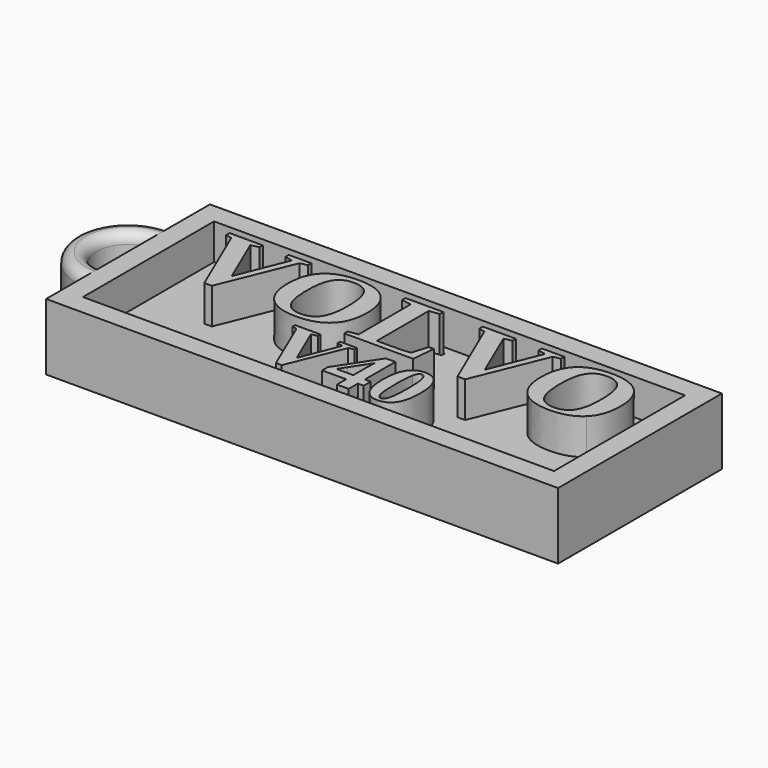
from build123d import *

# Parameters (mm, degrees)
F1_DEPTH = 3
F2_DEPTH = 3.5
F3_R     = 0.99999


# Not quite as in the source:
# - a fillet or chamfer is up to 0.001 mm smaller than in the source, because OpenCascade refuses the exact size


with BuildPart() as f1:
    # F0 (on Top) → F1 (new body)
    with BuildSketch(Plane.XY):
        Polygon((25, -10), (25, 10), (0, 10), (0, 8), (23, 8), (23, -8), (0, -8), (0, -10), align=None)
        Polygon((0, 8), (0, 10), (-25, 10), (-25, 5.1), (-25, 3.1), (-25, -3.1), (-25, -5.1), (-25, -10), (0, -10), (0, -8), (-23, -8), (-23, 8), align=None)
        with BuildLine():
            Line((23, 8), (0, 8))
            Line((0, 8), (0, 7.2330922616))
            Line((0, 7.2330922616), (0.1773994991, 7.2330922616))
            Line((0.1773994991, 7.2330922616), (0.1773994991, 6.8265888868))
            Line((0.1773994991, 6.8265888868), (0, 6.8041054881))
            Line((0, 6.8041054881), (0, 0.3510614427))
            Line((0, 0.3510614427), (0.544678864, 0.3510614427))
            add(Edge.make_bspline(
                [(0.544678864, 0.3510614427), (1.7320966167, 0.3510614427), (2.2901473023, 0.4633847436)],
                knots=[0, 0, 0, 1, 1, 1], degree=2))
            Line((2.2901473023, 0.4633847436), (2.7465721442, 2.0180818613))
            Line((2.7465721442, 2.0180818613), (3.2475697245, 2.0180818613))
            Line((3.2475697245, 2.0180818613), (3.0354034894, -0.2390816146))
            Line((3.0354034894, -0.2390816146), (0, -0.2390816146))
            Line((0, -0.2390816146), (0, -3.5619589872))
            Line((0, -3.5619589872), (1.3642210542, -1.4834557912))
            Line((1.3642210542, -1.4834557912), (2.2953560595, -1.4834557912))
            Line((2.2953560595, -1.4834557912), (2.2953560595, -5.197168661))
            Line((2.2953560595, -5.197168661), (2.861074711, -5.197168661))
            Line((2.861074711, -5.197168661), (2.861074711, -6.0646941529))
            Line((2.861074711, -6.0646941529), (2.2953560595, -6.0646941529))
            Line((2.2953560595, -6.0646941529), (2.2953560595, -7.1853043046))
            Line((2.2953560595, -7.1853043046), (1.1571517871, -7.1853043046))
            Line((1.1571517871, -7.1853043046), (1.1571517871, -6.0646941529))
            Line((1.1571517871, -6.0646941529), (0, -6.0646941529))
            Line((0, -6.0646941529), (0, -8))
            Line((0, -8), (23, -8))
            Line((23, -8), (23, 8))
        make_face()
        with BuildLine():
            add(Edge.make_bspline(
                [(6.5578701571, -2.1628595305), (7.0227609628, -2.9004592076), (7.0227609628, -4.3255829875)],
                knots=[0, 0, 0, 1, 1, 1], degree=2))
            add(Edge.make_bspline(
                [(7.0227609628, -4.3255829875), (7.0227609628, -7.2705681205), (5.1618443461, -7.2705681205)],
                knots=[0, 0, 0, 1, 1, 1], degree=2))
            add(Edge.make_bspline(
                [(5.1618443461, -7.2705681205), (4.2658975823, -7.2705681205), (3.8091271401, -6.5174044134)],
                knots=[0, 0, 0, 1, 1, 1], degree=2))
            add(Edge.make_bspline(
                [(3.8091271401, -6.5174044134), (3.3523566978, -5.7642407064), (3.3523566978, -4.3255829875)],
                knots=[0, 0, 0, 1, 1, 1], degree=2))
            add(Edge.make_bspline(
                [(3.3523566978, -4.3255829875), (3.3523566978, -2.9180533284), (3.8091271401, -2.1716565908)],
                knots=[0, 0, 0, 1, 1, 1], degree=2))
            add(Edge.make_bspline(
                [(3.8091271401, -2.1716565908), (4.2658975823, -1.4252598533), (5.1956791937, -1.4252598533)],
                knots=[0, 0, 0, 1, 1, 1], degree=2))
            add(Edge.make_bspline(
                [(5.1956791937, -1.4252598533), (6.0929793514, -1.4252598533), (6.5578701571, -2.1628595305)],
                knots=[0, 0, 0, 1, 1, 1], degree=2))
        make_face(mode=Mode.SUBTRACT)
        Polygon((9.6393004203, 7.2330922616), (11.8394107908, 7.2330922616), (11.8394107908, 6.8265888868), (11.131595704, 6.675041576), (8.2450651611, -0.4120238398), (7.5051577026, -0.4120238398), (4.4688627584, 6.675041576), (3.8555418771, 6.8265888868), (3.8555418771, 7.2330922616), (7.1040030564, 7.2330922616), (7.1040030564, 6.8265888868), (6.3284374071, 6.675041576), (8.4304877531, 1.7773890735), (10.3916882455, 6.675041576), (9.6393004203, 6.8265888868), align=None, mode=Mode.SUBTRACT)
        with BuildLine():
            add(Edge.make_bspline(
                [(13.5224773953, 0.6238466021), (12.5258309632, 1.5990981197), (12.5258309632, 3.5050284164)],
                knots=[0, 0, 0, 1, 1, 1], degree=2))
            add(Edge.make_bspline(
                [(12.5258309632, 3.5050284164), (12.5258309632, 7.3168890099), (16.4090079382, 7.3168890099)],
                knots=[0, 0, 0, 1, 1, 1], degree=2))
            add(Edge.make_bspline(
                [(16.4090079382, 7.3168890099), (18.3256356922, 7.3168890099), (19.3062359384, 6.3496605852)],
                knots=[0, 0, 0, 1, 1, 1], degree=2))
            add(Edge.make_bspline(
                [(19.3062359384, 6.3496605852), (20.2868361846, 5.3824321605), (20.2868361846, 3.5050284164)],
                knots=[0, 0, 0, 1, 1, 1], degree=2))
            add(Edge.make_bspline(
                [(20.2868361846, 3.5050284164), (20.2868361846, 1.6044468483), (19.2946470264, 0.6265209664)],
                knots=[0, 0, 0, 1, 1, 1], degree=2))
            add(Edge.make_bspline(
                [(19.2946470264, 0.6265209664), (18.3024578681, -0.3514049155), (16.4090079382, -0.3514049155)],
                knots=[0, 0, 0, 1, 1, 1], degree=2))
            add(Edge.make_bspline(
                [(16.4090079382, -0.3514049155), (14.5191238273, -0.3514049155), (13.5224773953, 0.6238466021)],
                knots=[0, 0, 0, 1, 1, 1], degree=2))
        make_face(mode=Mode.SUBTRACT)
        Polygon((0, 7.2330922616), (0, 8), (-23, 8), (-23, -8), (0, -8), (0, -6.0646941529), (-1.1896332408, -6.0646941529), (-1.1896332408, -5.3744632623), (0, -3.5619589872), (0, -0.2390816146), (-3.6897312901, -0.2390816146), (-3.6897312901, 0.1674217602), (-2.7305259583, 0.318969071), (-2.7305259583, 6.6803903046), (-3.6825996519, 6.8265888868), (-3.6825996519, 7.2330922616), align=None)
        Polygon((-3.0762643416, -1.513230457), (-1.4061762652, -1.513230457), (-1.4061762652, -1.8218042669), (-1.9434736447, -1.9368427487), (-4.1346183737, -7.3165835132), (-4.6962768435, -7.3165835132), (-7.0011066603, -1.9368427487), (-7.466674163, -1.8218042669), (-7.466674163, -1.513230457), (-5.0007904717, -1.513230457), (-5.0007904717, -1.8218042669), (-5.5895168195, -1.9368427487), (-3.9938654078, -5.6546158003), (-2.5051321145, -1.9368427487), (-3.0762643416, -1.8218042669), align=None, mode=Mode.SUBTRACT)
        Polygon((-15.0878719701, 7.2330922616), (-12.8877615995, 7.2330922616), (-12.8877615995, 6.8265888868), (-13.5955766863, 6.675041576), (-16.4821072293, -0.4120238398), (-17.2220146878, -0.4120238398), (-20.258309632, 6.675041576), (-20.8716305132, 6.8265888868), (-20.8716305132, 7.2330922616), (-17.623169334, 7.2330922616), (-17.623169334, 6.8265888868), (-18.3987349832, 6.675041576), (-16.2966846373, 1.7773890735), (-14.3354841448, 6.675041576), (-15.0878719701, 6.8265888868), align=None, mode=Mode.SUBTRACT)
        with BuildLine():
            add(Edge.make_bspline(
                [(-11.2046949951, 0.6238466021), (-12.2013414272, 1.5990981197), (-12.2013414272, 3.5050284164)],
                knots=[0, 0, 0, 1, 1, 1], degree=2))
            add(Edge.make_bspline(
                [(-12.2013414272, 3.5050284164), (-12.2013414272, 7.3168890099), (-8.3181644522, 7.3168890099)],
                knots=[0, 0, 0, 1, 1, 1], degree=2))
            add(Edge.make_bspline(
                [(-8.3181644522, 7.3168890099), (-6.4015366982, 7.3168890099), (-5.420936452, 6.3496605852)],
                knots=[0, 0, 0, 1, 1, 1], degree=2))
            add(Edge.make_bspline(
                [(-5.420936452, 6.3496605852), (-4.4403362058, 5.3824321605), (-4.4403362058, 3.5050284164)],
                knots=[0, 0, 0, 1, 1, 1], degree=2))
            add(Edge.make_bspline(
                [(-4.4403362058, 3.5050284164), (-4.4403362058, 1.6044468483), (-5.432525364, 0.6265209664)],
                knots=[0, 0, 0, 1, 1, 1], degree=2))
            add(Edge.make_bspline(
                [(-5.432525364, 0.6265209664), (-6.4247145222, -0.3514049155), (-8.3181644522, -0.3514049155)],
                knots=[0, 0, 0, 1, 1, 1], degree=2))
            add(Edge.make_bspline(
                [(-8.3181644522, -0.3514049155), (-10.2080485631, -0.3514049155), (-11.2046949951, 0.6238466021)],
                knots=[0, 0, 0, 1, 1, 1], degree=2))
        make_face(mode=Mode.SUBTRACT)
        with BuildLine():
            Line((-25, 3.1), (-25, 5.1))
            ThreePointArc((-25, 5.1), (-30.1, 0), (-25, -5.1))
            Line((-25, -5.1), (-25, -3.1))
            ThreePointArc((-25, -3.1), (-28.1, 0), (-25, 3.1))
        make_face()
        Polygon((0, 6.8041054881), (0, 7.2330922616), (-3.6825996519, 7.2330922616), (-3.6825996519, 6.8265888868), (-2.7305259583, 6.6803903046), (-2.7305259583, 0.318969071), (-3.6897312901, 0.1674217602), (-3.6897312901, -0.2390816146), (0, -0.2390816146), (0, 0.3510614427), (-0.9761429724, 0.3510614427), (-0.9761429724, 6.6803903046), align=None)
        Polygon((0, 0.3510614427), (0, 6.8041054881), (-0.9761429724, 6.6803903046), (-0.9761429724, 0.3510614427), align=None)
        Polygon((-1.1896332408, -6.0646941529), (0, -6.0646941529), (0, -5.197168661), (-0.488575199, -5.197168661), (0, -4.4515723469), (0, -3.5619589872), (-1.1896332408, -5.3744632623), align=None)
        with BuildLine():
            Line((0, -5.197168661), (0, -6.0646941529))
            Line((0, -6.0646941529), (1.1571517871, -6.0646941529))
            Line((1.1571517871, -6.0646941529), (1.1571517871, -7.1853043046))
            Line((1.1571517871, -7.1853043046), (2.2953560595, -7.1853043046))
            Line((2.2953560595, -7.1853043046), (2.2953560595, -6.0646941529))
            Line((2.2953560595, -6.0646941529), (2.861074711, -6.0646941529))
            Line((2.861074711, -6.0646941529), (2.861074711, -5.197168661))
            Line((2.861074711, -5.197168661), (2.2953560595, -5.197168661))
            Line((2.2953560595, -5.197168661), (2.2953560595, -1.4834557912))
            Line((2.2953560595, -1.4834557912), (1.3642210542, -1.4834557912))
            Line((1.3642210542, -1.4834557912), (0, -3.5619589872))
            Line((0, -3.5619589872), (0, -4.4515723469))
            Line((0, -4.4515723469), (1.1991069981, -2.6216600636))
            add(Edge.make_bspline(
                [(1.1571517871, -3.5189602213), (1.1571517871, -3.0452723552), (1.1991069981, -2.6216600636)],
                knots=[0, 0, 0, 1, 1, 1], degree=2))
            Line((1.1571517871, -3.5189602213), (1.1571517871, -5.197168661))
            Line((1.1571517871, -5.197168661), (0, -5.197168661))
        make_face()
        with BuildLine():
            Line((0.544678864, 0.3510614427), (0, 0.3510614427))
            Line((0, 0.3510614427), (0, -0.2390816146))
            Line((0, -0.2390816146), (3.0354034894, -0.2390816146))
            Line((3.0354034894, -0.2390816146), (3.2475697245, 2.0180818613))
            Line((3.2475697245, 2.0180818613), (2.7465721442, 2.0180818613))
            Line((2.7465721442, 2.0180818613), (2.2901473023, 0.4633847436))
            add(Edge.make_bspline(
                [(0.544678864, 0.3510614427), (1.7320966167, 0.3510614427), (2.2901473023, 0.4633847436)],
                knots=[0, 0, 0, 1, 1, 1], degree=2))
        make_face()
        Polygon((-0.488575199, -5.197168661), (0, -5.197168661), (0, -4.4515723469), align=None)
        with BuildLine():
            Line((0, -4.4515723469), (0, -5.197168661))
            Line((0, -5.197168661), (1.1571517871, -5.197168661))
            Line((1.1571517871, -5.197168661), (1.1571517871, -3.5189602213))
            add(Edge.make_bspline(
                [(1.1571517871, -3.5189602213), (1.1571517871, -3.0452723552), (1.1991069981, -2.6216600636)],
                knots=[0, 0, 0, 1, 1, 1], degree=2))
            Line((1.1991069981, -2.6216600636), (0, -4.4515723469))
        make_face()
        Polygon((-1.4061762652, -1.8218042669), (-1.4061762652, -1.513230457), (-3.0762643416, -1.513230457), (-3.0762643416, -1.8218042669), (-2.5051321145, -1.9368427487), (-3.9938654078, -5.6546158003), (-5.5895168195, -1.9368427487), (-5.0007904717, -1.8218042669), (-5.0007904717, -1.513230457), (-7.466674163, -1.513230457), (-7.466674163, -1.8218042669), (-7.0011066603, -1.9368427487), (-4.6962768435, -7.3165835132), (-4.1346183737, -7.3165835132), (-1.9434736447, -1.9368427487), align=None)
        with BuildLine():
            add(Edge.make_bspline(
                [(7.0227609628, -4.3255829875), (7.0227609628, -7.2705681205), (5.1618443461, -7.2705681205)],
                knots=[0, 0, 0, 1, 1, 1], degree=2))
            add(Edge.make_bspline(
                [(6.5578701571, -2.1628595305), (7.0227609628, -2.9004592076), (7.0227609628, -4.3255829875)],
                knots=[0, 0, 0, 1, 1, 1], degree=2))
            add(Edge.make_bspline(
                [(5.1956791937, -1.4252598533), (6.0929793514, -1.4252598533), (6.5578701571, -2.1628595305)],
                knots=[0, 0, 0, 1, 1, 1], degree=2))
            add(Edge.make_bspline(
                [(3.8091271401, -2.1716565908), (4.2658975823, -1.4252598533), (5.1956791937, -1.4252598533)],
                knots=[0, 0, 0, 1, 1, 1], degree=2))
            add(Edge.make_bspline(
                [(3.3523566978, -4.3255829875), (3.3523566978, -2.9180533284), (3.8091271401, -2.1716565908)],
                knots=[0, 0, 0, 1, 1, 1], degree=2))
            add(Edge.make_bspline(
                [(3.8091271401, -6.5174044134), (3.3523566978, -5.7642407064), (3.3523566978, -4.3255829875)],
                knots=[0, 0, 0, 1, 1, 1], degree=2))
            add(Edge.make_bspline(
                [(5.1618443461, -7.2705681205), (4.2658975823, -7.2705681205), (3.8091271401, -6.5174044134)],
                knots=[0, 0, 0, 1, 1, 1], degree=2))
        make_face()
        with BuildLine():
            add(Edge.make_bspline(
                [(5.7844055415, -4.3255829875), (5.7844055415, -3.0060239321), (5.6362089091, -2.4288014324)],
                knots=[0, 0, 0, 1, 1, 1], degree=2))
            add(Edge.make_bspline(
                [(5.6341788183, -6.2609362688), (5.7844055415, -5.6749167088), (5.7844055415, -4.3255829875)],
                knots=[0, 0, 0, 1, 1, 1], degree=2))
            add(Edge.make_bspline(
                [(5.1713181034, -6.8469558288), (5.483952095, -6.8469558288), (5.6341788183, -6.2609362688)],
                knots=[0, 0, 0, 1, 1, 1], degree=2))
            add(Edge.make_bspline(
                [(4.7260515094, -6.2758236018), (4.8613908997, -6.8469558288), (5.1713181034, -6.8469558288)],
                knots=[0, 0, 0, 1, 1, 1], degree=2))
            add(Edge.make_bspline(
                [(4.590712119, -4.3255829875), (4.590712119, -5.7046913747), (4.7260515094, -6.2758236018)],
                knots=[0, 0, 0, 1, 1, 1], degree=2))
            add(Edge.make_bspline(
                [(4.7240214185, -2.4098539178), (4.590712119, -2.9681289028), (4.590712119, -4.3255829875)],
                knots=[0, 0, 0, 1, 1, 1], degree=2))
            add(Edge.make_bspline(
                [(5.1713181034, -1.8515789328), (4.8573307179, -1.8515789328), (4.7240214185, -2.4098539178)],
                knots=[0, 0, 0, 1, 1, 1], degree=2))
            add(Edge.make_bspline(
                [(5.6362089091, -2.4288014324), (5.4880122768, -1.8515789328), (5.1713181034, -1.8515789328)],
                knots=[0, 0, 0, 1, 1, 1], degree=2))
        make_face(mode=Mode.SUBTRACT)
        with BuildLine():
            add(Edge.make_bspline(
                [(5.6341788183, -6.2609362688), (5.7844055415, -5.6749167088), (5.7844055415, -4.3255829875)],
                knots=[0, 0, 0, 1, 1, 1], degree=2))
            add(Edge.make_bspline(
                [(5.7844055415, -4.3255829875), (5.7844055415, -3.0060239321), (5.6362089091, -2.4288014324)],
                knots=[0, 0, 0, 1, 1, 1], degree=2))
            add(Edge.make_bspline(
                [(5.6362089091, -2.4288014324), (5.4880122768, -1.8515789328), (5.1713181034, -1.8515789328)],
                knots=[0, 0, 0, 1, 1, 1], degree=2))
            add(Edge.make_bspline(
                [(5.1713181034, -1.8515789328), (4.8573307179, -1.8515789328), (4.7240214185, -2.4098539178)],
                knots=[0, 0, 0, 1, 1, 1], degree=2))
            add(Edge.make_bspline(
                [(4.7240214185, -2.4098539178), (4.590712119, -2.9681289028), (4.590712119, -4.3255829875)],
                knots=[0, 0, 0, 1, 1, 1], degree=2))
            add(Edge.make_bspline(
                [(4.590712119, -4.3255829875), (4.590712119, -5.7046913747), (4.7260515094, -6.2758236018)],
                knots=[0, 0, 0, 1, 1, 1], degree=2))
            add(Edge.make_bspline(
                [(4.7260515094, -6.2758236018), (4.8613908997, -6.8469558288), (5.1713181034, -6.8469558288)],
                knots=[0, 0, 0, 1, 1, 1], degree=2))
            add(Edge.make_bspline(
                [(5.1713181034, -6.8469558288), (5.483952095, -6.8469558288), (5.6341788183, -6.2609362688)],
                knots=[0, 0, 0, 1, 1, 1], degree=2))
        make_face()
        Polygon((-12.8877615995, 6.8265888868), (-12.8877615995, 7.2330922616), (-15.0878719701, 7.2330922616), (-15.0878719701, 6.8265888868), (-14.3354841448, 6.675041576), (-16.2966846373, 1.7773890735), (-18.3987349832, 6.675041576), (-17.623169334, 6.8265888868), (-17.623169334, 7.2330922616), (-20.8716305132, 7.2330922616), (-20.8716305132, 6.8265888868), (-20.258309632, 6.675041576), (-17.2220146878, -0.4120238398), (-16.4821072293, -0.4120238398), (-13.5955766863, 6.675041576), align=None)
        with BuildLine():
            add(Edge.make_bspline(
                [(-12.2013414272, 3.5050284164), (-12.2013414272, 7.3168890099), (-8.3181644522, 7.3168890099)],
                knots=[0, 0, 0, 1, 1, 1], degree=2))
            add(Edge.make_bspline(
                [(-11.2046949951, 0.6238466021), (-12.2013414272, 1.5990981197), (-12.2013414272, 3.5050284164)],
                knots=[0, 0, 0, 1, 1, 1], degree=2))
            add(Edge.make_bspline(
                [(-8.3181644522, -0.3514049155), (-10.2080485631, -0.3514049155), (-11.2046949951, 0.6238466021)],
                knots=[0, 0, 0, 1, 1, 1], degree=2))
            add(Edge.make_bspline(
                [(-5.432525364, 0.6265209664), (-6.4247145222, -0.3514049155), (-8.3181644522, -0.3514049155)],
                knots=[0, 0, 0, 1, 1, 1], degree=2))
            add(Edge.make_bspline(
                [(-4.4403362058, 3.5050284164), (-4.4403362058, 1.6044468483), (-5.432525364, 0.6265209664)],
                knots=[0, 0, 0, 1, 1, 1], degree=2))
            add(Edge.make_bspline(
                [(-5.420936452, 6.3496605852), (-4.4403362058, 5.3824321605), (-4.4403362058, 3.5050284164)],
                knots=[0, 0, 0, 1, 1, 1], degree=2))
            add(Edge.make_bspline(
                [(-8.3181644522, 7.3168890099), (-6.4015366982, 7.3168890099), (-5.420936452, 6.3496605852)],
                knots=[0, 0, 0, 1, 1, 1], degree=2))
        make_face()
        with BuildLine():
            add(Edge.make_bspline(
                [(-10.3524642357, 3.5050284164), (-10.3524642357, 1.7274676065), (-9.8648384769, 0.9670566883)],
                knots=[0, 0, 0, 1, 1, 1], degree=2))
            add(Edge.make_bspline(
                [(-9.8648384769, 6.0126906824), (-10.3524642357, 5.2718917691), (-10.3524642357, 3.5050284164)],
                knots=[0, 0, 0, 1, 1, 1], degree=2))
            add(Edge.make_bspline(
                [(-8.3181644522, 6.7534895957), (-9.3772127181, 6.7534895957), (-9.8648384769, 6.0126906824)],
                knots=[0, 0, 0, 1, 1, 1], degree=2))
            add(Edge.make_bspline(
                [(-6.7786220656, 6.0126906824), (-7.2662478244, 6.7534895957), (-8.3181644522, 6.7534895957)],
                knots=[0, 0, 0, 1, 1, 1], degree=2))
            add(Edge.make_bspline(
                [(-6.2909963068, 3.5050284164), (-6.2909963068, 5.2718917691), (-6.7786220656, 6.0126906824)],
                knots=[0, 0, 0, 1, 1, 1], degree=2))
            add(Edge.make_bspline(
                [(-6.7786220656, 0.9697310526), (-6.2909963068, 1.7328163351), (-6.2909963068, 3.5050284164)],
                knots=[0, 0, 0, 1, 1, 1], degree=2))
            add(Edge.make_bspline(
                [(-8.3181644522, 0.2066457701), (-7.2662478244, 0.2066457701), (-6.7786220656, 0.9697310526)],
                knots=[0, 0, 0, 1, 1, 1], degree=2))
            add(Edge.make_bspline(
                [(-9.8648384769, 0.9670566883), (-9.3772127181, 0.2066457701), (-8.3181644522, 0.2066457701)],
                knots=[0, 0, 0, 1, 1, 1], degree=2))
        make_face(mode=Mode.SUBTRACT)
        with BuildLine():
            add(Edge.make_bspline(
                [(-9.8648384769, 6.0126906824), (-10.3524642357, 5.2718917691), (-10.3524642357, 3.5050284164)],
                knots=[0, 0, 0, 1, 1, 1], degree=2))
            add(Edge.make_bspline(
                [(-10.3524642357, 3.5050284164), (-10.3524642357, 1.7274676065), (-9.8648384769, 0.9670566883)],
                knots=[0, 0, 0, 1, 1, 1], degree=2))
            add(Edge.make_bspline(
                [(-9.8648384769, 0.9670566883), (-9.3772127181, 0.2066457701), (-8.3181644522, 0.2066457701)],
                knots=[0, 0, 0, 1, 1, 1], degree=2))
            add(Edge.make_bspline(
                [(-8.3181644522, 0.2066457701), (-7.2662478244, 0.2066457701), (-6.7786220656, 0.9697310526)],
                knots=[0, 0, 0, 1, 1, 1], degree=2))
            add(Edge.make_bspline(
                [(-6.7786220656, 0.9697310526), (-6.2909963068, 1.7328163351), (-6.2909963068, 3.5050284164)],
                knots=[0, 0, 0, 1, 1, 1], degree=2))
            add(Edge.make_bspline(
                [(-6.2909963068, 3.5050284164), (-6.2909963068, 5.2718917691), (-6.7786220656, 6.0126906824)],
                knots=[0, 0, 0, 1, 1, 1], degree=2))
            add(Edge.make_bspline(
                [(-6.7786220656, 6.0126906824), (-7.2662478244, 6.7534895957), (-8.3181644522, 6.7534895957)],
                knots=[0, 0, 0, 1, 1, 1], degree=2))
            add(Edge.make_bspline(
                [(-8.3181644522, 6.7534895957), (-9.3772127181, 6.7534895957), (-9.8648384769, 6.0126906824)],
                knots=[0, 0, 0, 1, 1, 1], degree=2))
        make_face()
        Polygon((11.8394107908, 6.8265888868), (11.8394107908, 7.2330922616), (9.6393004203, 7.2330922616), (9.6393004203, 6.8265888868), (10.3916882455, 6.675041576), (8.4304877531, 1.7773890735), (6.3284374071, 6.675041576), (7.1040030564, 6.8265888868), (7.1040030564, 7.2330922616), (3.8555418771, 7.2330922616), (3.8555418771, 6.8265888868), (4.4688627584, 6.675041576), (7.5051577026, -0.4120238398), (8.2450651611, -0.4120238398), (11.131595704, 6.675041576), align=None)
        with BuildLine():
            add(Edge.make_bspline(
                [(12.5258309632, 3.5050284164), (12.5258309632, 7.3168890099), (16.4090079382, 7.3168890099)],
                knots=[0, 0, 0, 1, 1, 1], degree=2))
            add(Edge.make_bspline(
                [(13.5224773953, 0.6238466021), (12.5258309632, 1.5990981197), (12.5258309632, 3.5050284164)],
                knots=[0, 0, 0, 1, 1, 1], degree=2))
            add(Edge.make_bspline(
                [(16.4090079382, -0.3514049155), (14.5191238273, -0.3514049155), (13.5224773953, 0.6238466021)],
                knots=[0, 0, 0, 1, 1, 1], degree=2))
            add(Edge.make_bspline(
                [(19.2946470264, 0.6265209664), (18.3024578681, -0.3514049155), (16.4090079382, -0.3514049155)],
                knots=[0, 0, 0, 1, 1, 1], degree=2))
            add(Edge.make_bspline(
                [(20.2868361846, 3.5050284164), (20.2868361846, 1.6044468483), (19.2946470264, 0.6265209664)],
                knots=[0, 0, 0, 1, 1, 1], degree=2))
            add(Edge.make_bspline(
                [(19.3062359384, 6.3496605852), (20.2868361846, 5.3824321605), (20.2868361846, 3.5050284164)],
                knots=[0, 0, 0, 1, 1, 1], degree=2))
            add(Edge.make_bspline(
                [(16.4090079382, 7.3168890099), (18.3256356922, 7.3168890099), (19.3062359384, 6.3496605852)],
                knots=[0, 0, 0, 1, 1, 1], degree=2))
        make_face()
        with BuildLine():
            add(Edge.make_bspline(
                [(14.3747081547, 3.5050284164), (14.3747081547, 1.7274676065), (14.8623339135, 0.9670566883)],
                knots=[0, 0, 0, 1, 1, 1], degree=2))
            add(Edge.make_bspline(
                [(14.8623339135, 6.0126906824), (14.3747081547, 5.2718917691), (14.3747081547, 3.5050284164)],
                knots=[0, 0, 0, 1, 1, 1], degree=2))
            add(Edge.make_bspline(
                [(16.4090079382, 6.7534895957), (15.3499596723, 6.7534895957), (14.8623339135, 6.0126906824)],
                knots=[0, 0, 0, 1, 1, 1], degree=2))
            add(Edge.make_bspline(
                [(17.9485503247, 6.0126906824), (17.4609245659, 6.7534895957), (16.4090079382, 6.7534895957)],
                knots=[0, 0, 0, 1, 1, 1], degree=2))
            add(Edge.make_bspline(
                [(18.4361760835, 3.5050284164), (18.4361760835, 5.2718917691), (17.9485503247, 6.0126906824)],
                knots=[0, 0, 0, 1, 1, 1], degree=2))
            add(Edge.make_bspline(
                [(17.9485503247, 0.9697310526), (18.4361760835, 1.7328163351), (18.4361760835, 3.5050284164)],
                knots=[0, 0, 0, 1, 1, 1], degree=2))
            add(Edge.make_bspline(
                [(16.4090079382, 0.2066457701), (17.4609245659, 0.2066457701), (17.9485503247, 0.9697310526)],
                knots=[0, 0, 0, 1, 1, 1], degree=2))
            add(Edge.make_bspline(
                [(14.8623339135, 0.9670566883), (15.3499596723, 0.2066457701), (16.4090079382, 0.2066457701)],
                knots=[0, 0, 0, 1, 1, 1], degree=2))
        make_face(mode=Mode.SUBTRACT)
        with BuildLine():
            add(Edge.make_bspline(
                [(14.8623339135, 6.0126906824), (14.3747081547, 5.2718917691), (14.3747081547, 3.5050284164)],
                knots=[0, 0, 0, 1, 1, 1], degree=2))
            add(Edge.make_bspline(
                [(14.3747081547, 3.5050284164), (14.3747081547, 1.7274676065), (14.8623339135, 0.9670566883)],
                knots=[0, 0, 0, 1, 1, 1], degree=2))
            add(Edge.make_bspline(
                [(14.8623339135, 0.9670566883), (15.3499596723, 0.2066457701), (16.4090079382, 0.2066457701)],
                knots=[0, 0, 0, 1, 1, 1], degree=2))
            add(Edge.make_bspline(
                [(16.4090079382, 0.2066457701), (17.4609245659, 0.2066457701), (17.9485503247, 0.9697310526)],
                knots=[0, 0, 0, 1, 1, 1], degree=2))
            add(Edge.make_bspline(
                [(17.9485503247, 0.9697310526), (18.4361760835, 1.7328163351), (18.4361760835, 3.5050284164)],
                knots=[0, 0, 0, 1, 1, 1], degree=2))
            add(Edge.make_bspline(
                [(18.4361760835, 3.5050284164), (18.4361760835, 5.2718917691), (17.9485503247, 6.0126906824)],
                knots=[0, 0, 0, 1, 1, 1], degree=2))
            add(Edge.make_bspline(
                [(17.9485503247, 6.0126906824), (17.4609245659, 6.7534895957), (16.4090079382, 6.7534895957)],
                knots=[0, 0, 0, 1, 1, 1], degree=2))
            add(Edge.make_bspline(
                [(16.4090079382, 6.7534895957), (15.3499596723, 6.7534895957), (14.8623339135, 6.0126906824)],
                knots=[0, 0, 0, 1, 1, 1], degree=2))
        make_face()
    extrude(amount=-F1_DEPTH)

    # F0 (on Top) → F2 (join)
    with BuildSketch(Plane.XY):
        Polygon((0, 8), (0, 10), (-25, 10), (-25, 5.1), (-25, 3.1), (-25, -3.1), (-25, -5.1), (-25, -10), (0, -10), (0, -8), (-23, -8), (-23, 8), align=None)
        with BuildLine():
            Line((-25, 3.1), (-25, 5.1))
            ThreePointArc((-25, 5.1), (-30.1, 0), (-25, -5.1))
            Line((-25, -5.1), (-25, -3.1))
            ThreePointArc((-25, -3.1), (-28.1, 0), (-25, 3.1))
        make_face()
        Polygon((25, -10), (25, 10), (0, 10), (0, 8), (23, 8), (23, -8), (0, -8), (0, -10), align=None)
        with BuildLine():
            add(Edge.make_bspline(
                [(12.5258309632, 3.5050284164), (12.5258309632, 7.3168890099), (16.4090079382, 7.3168890099)],
                knots=[0, 0, 0, 1, 1, 1], degree=2))
            add(Edge.make_bspline(
                [(13.5224773953, 0.6238466021), (12.5258309632, 1.5990981197), (12.5258309632, 3.5050284164)],
                knots=[0, 0, 0, 1, 1, 1], degree=2))
            add(Edge.make_bspline(
                [(16.4090079382, -0.3514049155), (14.5191238273, -0.3514049155), (13.5224773953, 0.6238466021)],
                knots=[0, 0, 0, 1, 1, 1], degree=2))
            add(Edge.make_bspline(
                [(19.2946470264, 0.6265209664), (18.3024578681, -0.3514049155), (16.4090079382, -0.3514049155)],
                knots=[0, 0, 0, 1, 1, 1], degree=2))
            add(Edge.make_bspline(
                [(20.2868361846, 3.5050284164), (20.2868361846, 1.6044468483), (19.2946470264, 0.6265209664)],
                knots=[0, 0, 0, 1, 1, 1], degree=2))
            add(Edge.make_bspline(
                [(19.3062359384, 6.3496605852), (20.2868361846, 5.3824321605), (20.2868361846, 3.5050284164)],
                knots=[0, 0, 0, 1, 1, 1], degree=2))
            add(Edge.make_bspline(
                [(16.4090079382, 7.3168890099), (18.3256356922, 7.3168890099), (19.3062359384, 6.3496605852)],
                knots=[0, 0, 0, 1, 1, 1], degree=2))
        make_face()
        with BuildLine():
            add(Edge.make_bspline(
                [(14.3747081547, 3.5050284164), (14.3747081547, 1.7274676065), (14.8623339135, 0.9670566883)],
                knots=[0, 0, 0, 1, 1, 1], degree=2))
            add(Edge.make_bspline(
                [(14.8623339135, 6.0126906824), (14.3747081547, 5.2718917691), (14.3747081547, 3.5050284164)],
                knots=[0, 0, 0, 1, 1, 1], degree=2))
            add(Edge.make_bspline(
                [(16.4090079382, 6.7534895957), (15.3499596723, 6.7534895957), (14.8623339135, 6.0126906824)],
                knots=[0, 0, 0, 1, 1, 1], degree=2))
            add(Edge.make_bspline(
                [(17.9485503247, 6.0126906824), (17.4609245659, 6.7534895957), (16.4090079382, 6.7534895957)],
                knots=[0, 0, 0, 1, 1, 1], degree=2))
            add(Edge.make_bspline(
                [(18.4361760835, 3.5050284164), (18.4361760835, 5.2718917691), (17.9485503247, 6.0126906824)],
                knots=[0, 0, 0, 1, 1, 1], degree=2))
            add(Edge.make_bspline(
                [(17.9485503247, 0.9697310526), (18.4361760835, 1.7328163351), (18.4361760835, 3.5050284164)],
                knots=[0, 0, 0, 1, 1, 1], degree=2))
            add(Edge.make_bspline(
                [(16.4090079382, 0.2066457701), (17.4609245659, 0.2066457701), (17.9485503247, 0.9697310526)],
                knots=[0, 0, 0, 1, 1, 1], degree=2))
            add(Edge.make_bspline(
                [(14.8623339135, 0.9670566883), (15.3499596723, 0.2066457701), (16.4090079382, 0.2066457701)],
                knots=[0, 0, 0, 1, 1, 1], degree=2))
        make_face(mode=Mode.SUBTRACT)
        Polygon((11.8394107908, 6.8265888868), (11.8394107908, 7.2330922616), (9.6393004203, 7.2330922616), (9.6393004203, 6.8265888868), (10.3916882455, 6.675041576), (8.4304877531, 1.7773890735), (6.3284374071, 6.675041576), (7.1040030564, 6.8265888868), (7.1040030564, 7.2330922616), (3.8555418771, 7.2330922616), (3.8555418771, 6.8265888868), (4.4688627584, 6.675041576), (7.5051577026, -0.4120238398), (8.2450651611, -0.4120238398), (11.131595704, 6.675041576), align=None)
        Polygon((0, 6.8041054881), (0, 7.2330922616), (-3.6825996519, 7.2330922616), (-3.6825996519, 6.8265888868), (-2.7305259583, 6.6803903046), (-2.7305259583, 0.318969071), (-3.6897312901, 0.1674217602), (-3.6897312901, -0.2390816146), (0, -0.2390816146), (0, 0.3510614427), (-0.9761429724, 0.3510614427), (-0.9761429724, 6.6803903046), align=None)
        with BuildLine():
            Line((0.544678864, 0.3510614427), (0, 0.3510614427))
            Line((0, 0.3510614427), (0, -0.2390816146))
            Line((0, -0.2390816146), (3.0354034894, -0.2390816146))
            Line((3.0354034894, -0.2390816146), (3.2475697245, 2.0180818613))
            Line((3.2475697245, 2.0180818613), (2.7465721442, 2.0180818613))
            Line((2.7465721442, 2.0180818613), (2.2901473023, 0.4633847436))
            add(Edge.make_bspline(
                [(0.544678864, 0.3510614427), (1.7320966167, 0.3510614427), (2.2901473023, 0.4633847436)],
                knots=[0, 0, 0, 1, 1, 1], degree=2))
        make_face()
        Polygon((-12.8877615995, 6.8265888868), (-12.8877615995, 7.2330922616), (-15.0878719701, 7.2330922616), (-15.0878719701, 6.8265888868), (-14.3354841448, 6.675041576), (-16.2966846373, 1.7773890735), (-18.3987349832, 6.675041576), (-17.623169334, 6.8265888868), (-17.623169334, 7.2330922616), (-20.8716305132, 7.2330922616), (-20.8716305132, 6.8265888868), (-20.258309632, 6.675041576), (-17.2220146878, -0.4120238398), (-16.4821072293, -0.4120238398), (-13.5955766863, 6.675041576), align=None)
        with BuildLine():
            add(Edge.make_bspline(
                [(-12.2013414272, 3.5050284164), (-12.2013414272, 7.3168890099), (-8.3181644522, 7.3168890099)],
                knots=[0, 0, 0, 1, 1, 1], degree=2))
            add(Edge.make_bspline(
                [(-11.2046949951, 0.6238466021), (-12.2013414272, 1.5990981197), (-12.2013414272, 3.5050284164)],
                knots=[0, 0, 0, 1, 1, 1], degree=2))
            add(Edge.make_bspline(
                [(-8.3181644522, -0.3514049155), (-10.2080485631, -0.3514049155), (-11.2046949951, 0.6238466021)],
                knots=[0, 0, 0, 1, 1, 1], degree=2))
            add(Edge.make_bspline(
                [(-5.432525364, 0.6265209664), (-6.4247145222, -0.3514049155), (-8.3181644522, -0.3514049155)],
                knots=[0, 0, 0, 1, 1, 1], degree=2))
            add(Edge.make_bspline(
                [(-4.4403362058, 3.5050284164), (-4.4403362058, 1.6044468483), (-5.432525364, 0.6265209664)],
                knots=[0, 0, 0, 1, 1, 1], degree=2))
            add(Edge.make_bspline(
                [(-5.420936452, 6.3496605852), (-4.4403362058, 5.3824321605), (-4.4403362058, 3.5050284164)],
                knots=[0, 0, 0, 1, 1, 1], degree=2))
            add(Edge.make_bspline(
                [(-8.3181644522, 7.3168890099), (-6.4015366982, 7.3168890099), (-5.420936452, 6.3496605852)],
                knots=[0, 0, 0, 1, 1, 1], degree=2))
        make_face()
        with BuildLine():
            add(Edge.make_bspline(
                [(-10.3524642357, 3.5050284164), (-10.3524642357, 1.7274676065), (-9.8648384769, 0.9670566883)],
                knots=[0, 0, 0, 1, 1, 1], degree=2))
            add(Edge.make_bspline(
                [(-9.8648384769, 6.0126906824), (-10.3524642357, 5.2718917691), (-10.3524642357, 3.5050284164)],
                knots=[0, 0, 0, 1, 1, 1], degree=2))
            add(Edge.make_bspline(
                [(-8.3181644522, 6.7534895957), (-9.3772127181, 6.7534895957), (-9.8648384769, 6.0126906824)],
                knots=[0, 0, 0, 1, 1, 1], degree=2))
            add(Edge.make_bspline(
                [(-6.7786220656, 6.0126906824), (-7.2662478244, 6.7534895957), (-8.3181644522, 6.7534895957)],
                knots=[0, 0, 0, 1, 1, 1], degree=2))
            add(Edge.make_bspline(
                [(-6.2909963068, 3.5050284164), (-6.2909963068, 5.2718917691), (-6.7786220656, 6.0126906824)],
                knots=[0, 0, 0, 1, 1, 1], degree=2))
            add(Edge.make_bspline(
                [(-6.7786220656, 0.9697310526), (-6.2909963068, 1.7328163351), (-6.2909963068, 3.5050284164)],
                knots=[0, 0, 0, 1, 1, 1], degree=2))
            add(Edge.make_bspline(
                [(-8.3181644522, 0.2066457701), (-7.2662478244, 0.2066457701), (-6.7786220656, 0.9697310526)],
                knots=[0, 0, 0, 1, 1, 1], degree=2))
            add(Edge.make_bspline(
                [(-9.8648384769, 0.9670566883), (-9.3772127181, 0.2066457701), (-8.3181644522, 0.2066457701)],
                knots=[0, 0, 0, 1, 1, 1], degree=2))
        make_face(mode=Mode.SUBTRACT)
        Polygon((-1.4061762652, -1.8218042669), (-1.4061762652, -1.513230457), (-3.0762643416, -1.513230457), (-3.0762643416, -1.8218042669), (-2.5051321145, -1.9368427487), (-3.9938654078, -5.6546158003), (-5.5895168195, -1.9368427487), (-5.0007904717, -1.8218042669), (-5.0007904717, -1.513230457), (-7.466674163, -1.513230457), (-7.466674163, -1.8218042669), (-7.0011066603, -1.9368427487), (-4.6962768435, -7.3165835132), (-4.1346183737, -7.3165835132), (-1.9434736447, -1.9368427487), align=None)
        with BuildLine():
            Line((0, -5.197168661), (0, -6.0646941529))
            Line((0, -6.0646941529), (1.1571517871, -6.0646941529))
            Line((1.1571517871, -6.0646941529), (1.1571517871, -7.1853043046))
            Line((1.1571517871, -7.1853043046), (2.2953560595, -7.1853043046))
            Line((2.2953560595, -7.1853043046), (2.2953560595, -6.0646941529))
            Line((2.2953560595, -6.0646941529), (2.861074711, -6.0646941529))
            Line((2.861074711, -6.0646941529), (2.861074711, -5.197168661))
            Line((2.861074711, -5.197168661), (2.2953560595, -5.197168661))
            Line((2.2953560595, -5.197168661), (2.2953560595, -1.4834557912))
            Line((2.2953560595, -1.4834557912), (1.3642210542, -1.4834557912))
            Line((1.3642210542, -1.4834557912), (0, -3.5619589872))
            Line((0, -3.5619589872), (0, -4.4515723469))
            Line((0, -4.4515723469), (1.1991069981, -2.6216600636))
            add(Edge.make_bspline(
                [(1.1571517871, -3.5189602213), (1.1571517871, -3.0452723552), (1.1991069981, -2.6216600636)],
                knots=[0, 0, 0, 1, 1, 1], degree=2))
            Line((1.1571517871, -3.5189602213), (1.1571517871, -5.197168661))
            Line((1.1571517871, -5.197168661), (0, -5.197168661))
        make_face()
        with BuildLine():
            add(Edge.make_bspline(
                [(7.0227609628, -4.3255829875), (7.0227609628, -7.2705681205), (5.1618443461, -7.2705681205)],
                knots=[0, 0, 0, 1, 1, 1], degree=2))
            add(Edge.make_bspline(
                [(6.5578701571, -2.1628595305), (7.0227609628, -2.9004592076), (7.0227609628, -4.3255829875)],
                knots=[0, 0, 0, 1, 1, 1], degree=2))
            add(Edge.make_bspline(
                [(5.1956791937, -1.4252598533), (6.0929793514, -1.4252598533), (6.5578701571, -2.1628595305)],
                knots=[0, 0, 0, 1, 1, 1], degree=2))
            add(Edge.make_bspline(
                [(3.8091271401, -2.1716565908), (4.2658975823, -1.4252598533), (5.1956791937, -1.4252598533)],
                knots=[0, 0, 0, 1, 1, 1], degree=2))
            add(Edge.make_bspline(
                [(3.3523566978, -4.3255829875), (3.3523566978, -2.9180533284), (3.8091271401, -2.1716565908)],
                knots=[0, 0, 0, 1, 1, 1], degree=2))
            add(Edge.make_bspline(
                [(3.8091271401, -6.5174044134), (3.3523566978, -5.7642407064), (3.3523566978, -4.3255829875)],
                knots=[0, 0, 0, 1, 1, 1], degree=2))
            add(Edge.make_bspline(
                [(5.1618443461, -7.2705681205), (4.2658975823, -7.2705681205), (3.8091271401, -6.5174044134)],
                knots=[0, 0, 0, 1, 1, 1], degree=2))
        make_face()
        with BuildLine():
            add(Edge.make_bspline(
                [(5.7844055415, -4.3255829875), (5.7844055415, -3.0060239321), (5.6362089091, -2.4288014324)],
                knots=[0, 0, 0, 1, 1, 1], degree=2))
            add(Edge.make_bspline(
                [(5.6341788183, -6.2609362688), (5.7844055415, -5.6749167088), (5.7844055415, -4.3255829875)],
                knots=[0, 0, 0, 1, 1, 1], degree=2))
            add(Edge.make_bspline(
                [(5.1713181034, -6.8469558288), (5.483952095, -6.8469558288), (5.6341788183, -6.2609362688)],
                knots=[0, 0, 0, 1, 1, 1], degree=2))
            add(Edge.make_bspline(
                [(4.7260515094, -6.2758236018), (4.8613908997, -6.8469558288), (5.1713181034, -6.8469558288)],
                knots=[0, 0, 0, 1, 1, 1], degree=2))
            add(Edge.make_bspline(
                [(4.590712119, -4.3255829875), (4.590712119, -5.7046913747), (4.7260515094, -6.2758236018)],
                knots=[0, 0, 0, 1, 1, 1], degree=2))
            add(Edge.make_bspline(
                [(4.7240214185, -2.4098539178), (4.590712119, -2.9681289028), (4.590712119, -4.3255829875)],
                knots=[0, 0, 0, 1, 1, 1], degree=2))
            add(Edge.make_bspline(
                [(5.1713181034, -1.8515789328), (4.8573307179, -1.8515789328), (4.7240214185, -2.4098539178)],
                knots=[0, 0, 0, 1, 1, 1], degree=2))
            add(Edge.make_bspline(
                [(5.6362089091, -2.4288014324), (5.4880122768, -1.8515789328), (5.1713181034, -1.8515789328)],
                knots=[0, 0, 0, 1, 1, 1], degree=2))
        make_face(mode=Mode.SUBTRACT)
        Polygon((-1.1896332408, -6.0646941529), (0, -6.0646941529), (0, -5.197168661), (-0.488575199, -5.197168661), (0, -4.4515723469), (0, -3.5619589872), (-1.1896332408, -5.3744632623), align=None)
    extrude(amount=F2_DEPTH)

    # F3 (radius 1 in the source; OpenCascade refuses exactly that, so slightly less here)
    f3_edges = [f1.edges().sort_by_distance(p)[0] for p in [
        (-28.1, 0, 3.5),
        (-30.1, 0, 3.5),
        (-30.1, 0, -3),
        (-28.1, 0, -3),
    ]]
    fillet(f3_edges, radius=F3_R)


solid = f1.part
